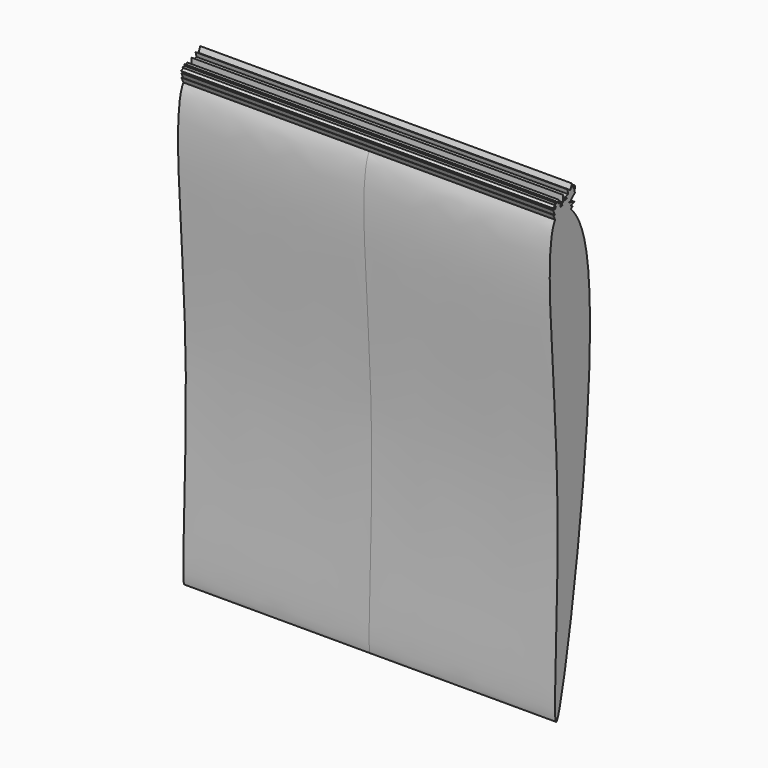
from build123d import *

# Parameters (mm, degrees)
F1_DEPTH = 63.5


with BuildPart() as f1:
    # F0 (on Right) → F1 (new body, symmetric)
    with BuildSketch(Plane.YZ):
        with BuildLine():
            add(Edge.make_bspline(
                [(-2.5031952433, 74.8461923193), (-2.3533415993, 75.0276387666), (-2.1963644561, 75.1912104401), (-2.0320170307, 75.336497153)],
                knots=[0.9934294222, 0.9934294222, 0.9934294222, 0.9934294222, 1, 1, 1, 1], degree=3))
            add(Edge.make_bspline(
                [(-2.0320170307, 75.336497153), (-1.8891955809, 75.4627544334), (-1.7408081058, 75.5752029408), (-1.5873915563, 75.6737167739)],
                knots=[0, 0, 0, 0, 0.0057099735, 0.0057099735, 0.0057099735, 0.0057099735], degree=3))
            Line((-1.5873915563, 75.6737167739), (-2.3197238782, 75.9019267209))
            Line((-2.3197238782, 75.9019267209), (-3.0087709391, 75.537379435))
            Line((-3.0087709391, 75.537379435), (-3.3884674872, 75.336497153))
            Line((-3.3884674872, 75.336497153), (-2.5031952433, 74.8461923193))
        make_face()
        with BuildLine():
            add(Edge.make_bspline(
                [(-2.0320170307, 75.336497153), (-1.8891955809, 75.4627544334), (-1.7408081058, 75.5752029408), (-1.5873915563, 75.6737167739)],
                knots=[0, 0, 0, 0, 0.0057099735, 0.0057099735, 0.0057099735, 0.0057099735], degree=3))
            add(Edge.make_bspline(
                [(-2.5031952433, 74.8461923193), (-2.3533415993, 75.0276387666), (-2.1963644561, 75.1912104401), (-2.0320170307, 75.336497153)],
                knots=[0.9934294222, 0.9934294222, 0.9934294222, 0.9934294222, 1, 1, 1, 1], degree=3))
            Line((-2.5031952433, 74.8461923193), (-2.981348253, 74.1680218189))
            add(Edge.make_bspline(
                [(5.280060228, 72.8526241439), (7.0114055785, 70.5658194338), (19.9534117553, 42.5855454276), (-9.4568688164, -135.9427321675), (2.3047634441, -4.9873481871), (-8.3046344498, 65.3969700213), (-2.981348253, 74.1680218189)],
                knots=[0.0751955785, 0.0751955785, 0.0751955785, 0.0751955785, 0.1255570674, 0.4789595318, 0.7253581944, 0.9860523361, 0.9860523361, 0.9860523361, 0.9860523361], degree=3))
            add(Edge.make_bspline(
                [(4.558134096, 73.7302112384), (4.8003585227, 73.4604084562), (5.0413225391, 73.1679549189), (5.280060228, 72.8526241439)],
                knots=[0.0682511607, 0.0682511607, 0.0682511607, 0.0682511607, 0.0751955785, 0.0751955785, 0.0751955785, 0.0751955785], degree=3))
            add(Edge.make_bspline(
                [(4.1172295334, 74.1951779468), (4.264516573, 74.048449974), (4.4115561068, 73.8934778), (4.558134096, 73.7302112384)],
                knots=[0.0640488644, 0.0640488644, 0.0640488644, 0.0640488644, 0.0682511607, 0.0682511607, 0.0682511607, 0.0682511607], degree=3))
            add(Edge.make_bspline(
                [(3.6763249708, 74.609368014), (3.8233977451, 74.4794605202), (3.9704365633, 74.3414137255), (4.1172295334, 74.1951779468)],
                knots=[0.0598606647, 0.0598606647, 0.0598606647, 0.0598606647, 0.0640488644, 0.0640488644, 0.0640488644, 0.0640488644], degree=3))
            add(Edge.make_bspline(
                [(2.0872520516, 75.7028253852), (2.6106797609, 75.4435060137), (3.1437250175, 75.0798067166), (3.6763249708, 74.609368014)],
                knots=[0.0446937854, 0.0446937854, 0.0446937854, 0.0446937854, 0.0598606647, 0.0598606647, 0.0598606647, 0.0598606647], degree=3))
            Line((2.0872520516, 75.7028253852), (0.9867487565, 76.098998544))
            add(Edge.make_bspline(
                [(-0.3830142642, 76.1440130478), (0.0531822749, 76.2183929611), (0.5125534467, 76.2040407853), (0.9867487565, 76.098998544)],
                knots=[0.0196351754, 0.0196351754, 0.0196351754, 0.0196351754, 0.0338877489, 0.0338877489, 0.0338877489, 0.0338877489], degree=3))
            Line((-0.3830142642, 76.1440130478), (-1.5873915563, 75.6737167739))
        make_face()
        with BuildLine():
            Line((-2.2569033628, 77.1257479092), (-1.5873915563, 75.6737167739))
            add(Edge.make_bspline(
                [(-1.5873915563, 75.6737167739), (-1.2132468387, 75.9139674535), (-0.8091916762, 76.0713415886), (-0.3830142642, 76.1440130478)],
                knots=[0.0057099735, 0.0057099735, 0.0057099735, 0.0057099735, 0.0196351754, 0.0196351754, 0.0196351754, 0.0196351754], degree=3))
            Line((-0.3830142642, 76.1440130478), (-0.6890374261, 76.8008807945))
            Line((-0.6890374261, 76.8008807945), (-1.4403613131, 78.4135705847))
            Line((-1.4403613131, 78.4135705847), (-1.6477123366, 78.8586421238))
            Line((-1.6477123366, 78.8586421238), (-2.2407262096, 78.5852114929))
            Line((-2.2407262096, 78.5852114929), (-2.1511793417, 78.3231779933))
            Line((-2.1511793417, 78.3231779933), (-2.5002173073, 78.4655636773))
            Line((-2.5002173073, 78.4655636773), (-2.8090220876, 78.3231779933))
            Line((-2.8090220876, 78.3231779933), (-2.6694845793, 78.0205503106))
            Line((-2.6694845793, 78.0205503106), (-2.2899973688, 77.1975218893))
            Line((-2.2899973688, 77.1975218893), (-2.1982068219, 77.239845262))
            Line((-2.1982068219, 77.239845262), (-2.2569033628, 77.1257479092))
        make_face()
        Polygon((-2.3197238782, 75.9019267209), (-1.5873915563, 75.6737167739), (-2.2569033628, 77.1257479092), (-2.8081836648, 76.0541409256), align=None)
        with BuildLine():
            add(Edge.make_bspline(
                [(-1.5873915563, 75.6737167739), (-1.2132468387, 75.9139674535), (-0.8091916762, 76.0713415886), (-0.3830142642, 76.1440130478)],
                knots=[0.0057099735, 0.0057099735, 0.0057099735, 0.0057099735, 0.0196351754, 0.0196351754, 0.0196351754, 0.0196351754], degree=3))
            Line((-1.5873915563, 75.6737167739), (-0.3830142642, 76.1440130478))
        make_face()
        with BuildLine():
            Line((-2.981348253, 74.1680218189), (-2.5031952433, 74.8461923193))
            add(Edge.make_bspline(
                [(-2.981348253, 74.1680218189), (-2.8307106495, 74.416223808), (-2.6714427358, 74.6424741518), (-2.5031952433, 74.8461923193)],
                knots=[0.9860523361, 0.9860523361, 0.9860523361, 0.9860523361, 0.9934294222, 0.9934294222, 0.9934294222, 0.9934294222], degree=3))
        make_face()
        with BuildLine():
            add(Edge.make_bspline(
                [(-2.981348253, 74.1680218189), (-2.8307106495, 74.416223808), (-2.6714427358, 74.6424741518), (-2.5031952433, 74.8461923193)],
                knots=[0.9860523361, 0.9860523361, 0.9860523361, 0.9860523361, 0.9934294222, 0.9934294222, 0.9934294222, 0.9934294222], degree=3))
            Line((-2.5031952433, 74.8461923193), (-3.3884674872, 75.336497153))
            Line((-3.3884674872, 75.336497153), (-3.0087709391, 75.537379435))
            Line((-3.0087709391, 75.537379435), (-3.817089441, 75.9805697295))
            Line((-3.817089441, 75.9805697295), (-2.981348253, 74.1680218189))
        make_face()
        with BuildLine():
            Line((-0.6890374261, 76.8008807945), (-0.3830142642, 76.1440130478))
            add(Edge.make_bspline(
                [(-0.3830142642, 76.1440130478), (0.0531822749, 76.2183929611), (0.5125534467, 76.2040407853), (0.9867487565, 76.098998544)],
                knots=[0.0196351754, 0.0196351754, 0.0196351754, 0.0196351754, 0.0338877489, 0.0338877489, 0.0338877489, 0.0338877489], degree=3))
            Line((0.9867487565, 76.098998544), (0.7385915378, 76.1883333325))
            Line((0.7385915378, 76.1883333325), (2.0733734483, 78.5983552125))
            Line((2.0733734483, 78.5983552125), (1.1083647041, 78.2685748189))
            Line((1.1083647041, 78.2685748189), (0.3825913591, 78.0205503106))
            Line((0.3825913591, 78.0205503106), (-0.2254049465, 78.2685748189))
            Line((-0.2254049465, 78.2685748189), (0.1438712369, 77.187992853))
            Line((0.1438712369, 77.187992853), (-0.4348183983, 77.4240620708))
            Line((-0.4348183983, 77.4240620708), (-0.6890374261, 76.8008807945))
        make_face()
        Polygon((-2.8081836648, 76.0541409256), (-2.2569033628, 77.1257479092), (-2.2899973688, 77.1975218893), (-3.4018163569, 76.6848772764), (-3.0356504681, 77.3527137935), (-3.8457969204, 77.3527137935), (-3.0087709391, 75.537379435), (-2.3197238782, 75.9019267209), align=None)
        Polygon((-2.2899973688, 77.1975218893), (-2.2569033628, 77.1257479092), (-2.1982068219, 77.239845262), align=None)
        with BuildLine():
            Line((0.7385915378, 76.1883333325), (0.9867487565, 76.098998544))
            add(Edge.make_bspline(
                [(0.9867487565, 76.098998544), (1.3462748329, 76.0193574676), (1.7143224031, 75.8875841978), (2.0872520516, 75.7028253852)],
                knots=[0.0338877489, 0.0338877489, 0.0338877489, 0.0338877489, 0.0446937854, 0.0446937854, 0.0446937854, 0.0446937854], degree=3))
            Line((2.0872520516, 75.7028253852), (2.8149356255, 77.0166979519))
            Line((2.8149356255, 77.0166979519), (3.1620607729, 77.6434514267))
            Line((3.1620607729, 77.6434514267), (4.059301739, 79.2634691559))
            Line((4.059301739, 79.2634691559), (4.2368694943, 79.5840774682))
            Line((4.2368694943, 79.5840774682), (2.9990179464, 80.2696570754))
            Line((2.9990179464, 80.2696570754), (2.619312158, 79.5840774682))
            Line((2.619312158, 79.5840774682), (2.0733734483, 78.5983552125))
            Line((2.0733734483, 78.5983552125), (0.7385915378, 76.1883333325))
        make_face()
        with BuildLine():
            add(Edge.make_bspline(
                [(0.9867487565, 76.098998544), (1.3462748329, 76.0193574676), (1.7143224031, 75.8875841978), (2.0872520516, 75.7028253852)],
                knots=[0.0338877489, 0.0338877489, 0.0338877489, 0.0338877489, 0.0446937854, 0.0446937854, 0.0446937854, 0.0446937854], degree=3))
            Line((0.9867487565, 76.098998544), (2.0872520516, 75.7028253852))
        make_face()
        Polygon((-1.4403613131, 78.4135705847), (-0.6890374261, 76.8008807945), (-0.5820615334, 78.3544704318), (-1.0112114232, 78.3840205083), align=None)
        Polygon((-3.4018163569, 76.6848772764), (-2.2899973688, 77.1975218893), (-2.6694845793, 78.0205503106), (-3.0356504681, 77.3527137935), align=None)
        with BuildLine():
            Line((3.6763249708, 76.1440130478), (2.0872520516, 75.7028253852))
            add(Edge.make_bspline(
                [(2.0872520516, 75.7028253852), (2.6106797609, 75.4435060137), (3.1437250175, 75.0798067166), (3.6763249708, 74.609368014)],
                knots=[0.0446937854, 0.0446937854, 0.0446937854, 0.0446937854, 0.0598606647, 0.0598606647, 0.0598606647, 0.0598606647], degree=3))
            Line((3.6763249708, 74.609368014), (3.6763249708, 75.7028253852))
            Line((3.6763249708, 75.7028253852), (3.6763249708, 76.1440130478))
        make_face()
        Polygon((2.8149356255, 77.0166979519), (2.0872520516, 75.7028253852), (3.6763249708, 76.1440130478), (3.6763249708, 75.7028253852), (5.280060228, 76.2396529317), (4.3258606793, 76.5404312399), align=None)
        Polygon((-1.0112114232, 79.1521631181), (-1.4403613131, 78.4135705847), (-1.0112114232, 78.3840205083), align=None)
        Polygon((-1.6477123366, 78.8586421238), (-1.4403613131, 78.4135705847), (-1.4403613131, 79.5840774682), (-1.8421410574, 78.8586421238), (-2.5820769138, 79.5840774682), (-2.3341679132, 78.8586421238), (-2.2407262096, 78.5852114929), align=None)
        Polygon((-3.9583467878, 78.0205503106), (-2.6694845793, 78.0205503106), (-2.8090220876, 78.3231779933), (-2.5002173073, 78.4655636773), (-2.832915338, 78.6012836886), align=None)
        Polygon((3.6763249708, 75.7028253852), (3.6763249708, 74.609368014), (4.558134096, 75.2144385873), align=None)
        Polygon((3.1620607729, 77.6434514267), (2.8149356255, 77.0166979519), (4.2936985152, 77.0166979519), (3.7278796441, 77.3300746893), (3.6735305559, 77.3601757354), align=None)
        Polygon((0.9867440243, 79.2001809928), (2.0733734483, 78.5983552125), (2.619312158, 79.5840774682), align=None)
        Polygon((4.059301739, 79.2634691559), (3.1620607729, 77.6434514267), (3.6735305559, 77.3601757354), (3.7591097802, 77.3580947163), (5.0101839906, 78.4805724743), align=None)
        Polygon((2.2468396386, 81.1680637901), (2.619312158, 79.5840774682), (2.9990179464, 80.2696570754), (4.2368694943, 79.5840774682), (4.9254237576, 80.2863950385), (4.6729080744, 80.9793676024), (4.2368694943, 82.1759775281), (3.534725517, 80.4547728496), align=None)
        Polygon((0.3825913591, 78.0205503106), (1.1083647041, 78.2685748189), (0.4196934169, 80.2837759256), align=None)
        Polygon((-2.1511793417, 78.3231779933), (-2.2407262096, 78.5852114929), (-2.5002173073, 78.4655636773), align=None)
        Polygon((-2.5002173073, 78.4655636773), (-2.2407262096, 78.5852114929), (-2.3341679132, 78.8586421238), (-2.832915338, 78.6012836886), align=None)
        Polygon((-3.4637924188, 78.8586421238), (-2.832915338, 78.6012836886), (-2.3341679132, 78.8586421238), align=None)
        Polygon((4.2368694943, 79.5840774682), (4.059301739, 79.2634691559), (5.0101839906, 78.4805724743), (5.6139780208, 79.0223032236), (5.2050605226, 79.1891160159), align=None)
        Polygon((4.9254237576, 80.2863950385), (4.2368694943, 79.5840774682), (5.2050605226, 79.1891160159), (5.6139780208, 80.9887126088), (5.2903378525, 80.6586032931), align=None)
    extrude(amount=F1_DEPTH, both=True)


with BuildPart() as f1b:
    # F0 (on Right) → F1, piece 2 (new body, symmetric)
    with BuildSketch(Plane.YZ):
        Polygon((3.7591097802, 77.3580947163), (3.7278796441, 77.3300746893), (3.8055084945, 77.3569664447), align=None)
    extrude(amount=F1_DEPTH, both=True)


solid = Compound([f1.part, f1b.part])
